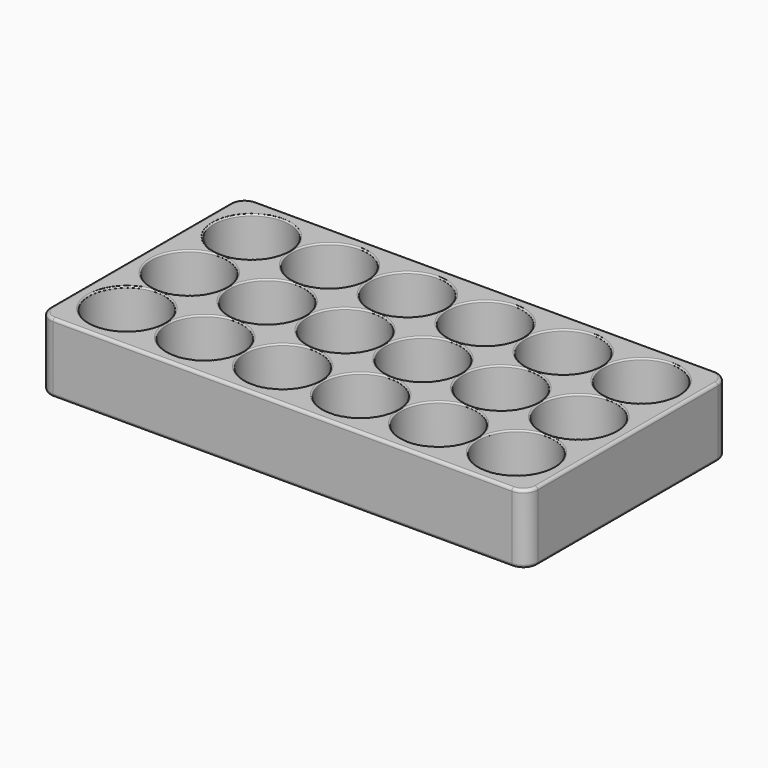
from build123d import *

# Parameters (mm, degrees)
F0_W         = 169
F0_H         = 88
F0_R         = 13.1
F1_DEPTH     = 22
F2_W         = 169
F2_H         = 88
F3_DEPTH     = 2
F4_R         = 1
F6_T1_DEPTH  = 24
F6_T4_ANGLE  = 90
F6_T6_ANGLE  = 90
F6_T8_ANGLE  = 90
F6_T10_ANGLE = 90
F6_T12_ANGLE = 90
F6_T14_ANGLE = 90
F6_T16_ANGLE = 90
F6_T18_ANGLE = 90


# Not quite as in the source:
# - a fillet or chamfer that OpenCascade refuses, or shapes differently, is made with other operations: its cross-section is extruded or revolved along the edge and cut away or added


with BuildPart() as f1:
    # F0 (on Top) → F1 (new body)
    with BuildSketch(Plane.XY):
        with Locations((67.5, 27)):
            Rectangle(F0_W, F0_H)
        Circle(F0_R, mode=Mode.SUBTRACT)
        with Locations((27, 0)):
            Circle(F0_R, mode=Mode.SUBTRACT)
        with Locations((54, 0)):
            Circle(F0_R, mode=Mode.SUBTRACT)
        with Locations((81, 0)):
            Circle(F0_R, mode=Mode.SUBTRACT)
        with Locations((108, 0)):
            Circle(F0_R, mode=Mode.SUBTRACT)
        with Locations((135, 0)):
            Circle(F0_R, mode=Mode.SUBTRACT)
        with Locations((0, 27)):
            Circle(F0_R, mode=Mode.SUBTRACT)
        with Locations((27, 27)):
            Circle(F0_R, mode=Mode.SUBTRACT)
        with Locations((54, 27)):
            Circle(F0_R, mode=Mode.SUBTRACT)
        with Locations((0, 54)):
            Circle(F0_R, mode=Mode.SUBTRACT)
        with Locations((27, 54)):
            Circle(F0_R, mode=Mode.SUBTRACT)
        with Locations((54, 54)):
            Circle(F0_R, mode=Mode.SUBTRACT)
        with Locations((81, 27)):
            Circle(F0_R, mode=Mode.SUBTRACT)
        with Locations((108, 27)):
            Circle(F0_R, mode=Mode.SUBTRACT)
        with Locations((135, 27)):
            Circle(F0_R, mode=Mode.SUBTRACT)
        with Locations((81, 54)):
            Circle(F0_R, mode=Mode.SUBTRACT)
        with Locations((108, 54)):
            Circle(F0_R, mode=Mode.SUBTRACT)
        with Locations((135, 54)):
            Circle(F0_R, mode=Mode.SUBTRACT)
    extrude(amount=-F1_DEPTH)

    # F2 (on face) → F3 (join)
    with BuildSketch(Plane(origin=(0, 0, -22), x_dir=(1, 0, 0), z_dir=(0, 0, -1))):
        with Locations((67.5, -27)):
            Rectangle(F2_W, F2_H)
    extrude(amount=F3_DEPTH)

    # F4
    f4_edges = [f1.edges().sort_by_distance(p)[0] for p in [
        (-17, 27, 0),
        (67.5, 71, 0),
        (152, 27, 0),
        (67.5, -17, 0),
        (67.5, 71, -24),
        (152, 27, -24),
        (67.5, -17, -24),
        (-17, 27, -24),
    ]]
    fillet(f4_edges, radius=F4_R)

    # F5: fillet of radius 0.5 on 22 edges, made by hand

    # F5_s1 → F5_t2 (revolve, cut)
    with BuildSketch(Plane.XZ):
        with BuildLine():
            ThreePointArc((148.6, 0), (148.2464466094, -0.1464466094), (148.1, -0.5))
            Line((148.1, -0.5), (148.1, 0))
            Line((148.1, 0), (148.6, 0))
        make_face()
    revolve(axis=Axis((135, 0, 0), (0, 0, 1)), mode=Mode.SUBTRACT)

    # F5_s3 → F5_t4 (revolve, cut)
    with BuildSketch(Plane.XZ):
        with BuildLine():
            ThreePointArc((13.6, 0), (13.2464466094, -0.1464466094), (13.1, -0.5))
            Line((13.1, -0.5), (13.1, 0))
            Line((13.1, 0), (13.6, 0))
        make_face()
    revolve(axis=Axis((0, 0, 0), (0, 0, 1)), mode=Mode.SUBTRACT)

    # F5_s5 → F5_t6 (revolve, cut)
    with BuildSketch(Plane.XZ):
        with BuildLine():
            ThreePointArc((40.6, 0), (40.2464466094, -0.1464466094), (40.1, -0.5))
            Line((40.1, -0.5), (40.1, 0))
            Line((40.1, 0), (40.6, 0))
        make_face()
    revolve(axis=Axis((27, 0, 0), (0, 0, 1)), mode=Mode.SUBTRACT)

    # F5_s7 → F5_t8 (revolve, cut)
    with BuildSketch(Plane.XZ):
        with BuildLine():
            ThreePointArc((67.6, 0), (67.2464466094, -0.1464466094), (67.1, -0.5))
            Line((67.1, -0.5), (67.1, 0))
            Line((67.1, 0), (67.6, 0))
        make_face()
    revolve(axis=Axis((54, 0, 0), (0, 0, 1)), mode=Mode.SUBTRACT)

    # F5_s9 → F5_t10 (revolve, cut)
    with BuildSketch(Plane.XZ):
        with BuildLine():
            ThreePointArc((94.6, 0), (94.2464466094, -0.1464466094), (94.1, -0.5))
            Line((94.1, -0.5), (94.1, 0))
            Line((94.1, 0), (94.6, 0))
        make_face()
    revolve(axis=Axis((81, 0, 0), (0, 0, 1)), mode=Mode.SUBTRACT)

    # F5_s11 → F5_t12 (revolve, cut)
    with BuildSketch(Plane.XZ):
        with BuildLine():
            ThreePointArc((121.6, 0), (121.2464466094, -0.1464466094), (121.1, -0.5))
            Line((121.1, -0.5), (121.1, 0))
            Line((121.1, 0), (121.6, 0))
        make_face()
    revolve(axis=Axis((108, 0, 0), (0, 0, 1)), mode=Mode.SUBTRACT)

    # F5_s13 → F5_t14 (revolve, cut)
    with BuildSketch(Plane.XZ.offset(-27)):
        with BuildLine():
            ThreePointArc((13.6, 0), (13.2464466094, -0.1464466094), (13.1, -0.5))
            Line((13.1, -0.5), (13.1, 0))
            Line((13.1, 0), (13.6, 0))
        make_face()
    revolve(axis=Axis((0, 27, 0), (0, 0, 1)), mode=Mode.SUBTRACT)

    # F5_s15 → F5_t16 (revolve, cut)
    with BuildSketch(Plane.XZ.offset(-27)):
        with BuildLine():
            ThreePointArc((40.6, 0), (40.2464466094, -0.1464466094), (40.1, -0.5))
            Line((40.1, -0.5), (40.1, 0))
            Line((40.1, 0), (40.6, 0))
        make_face()
    revolve(axis=Axis((27, 27, 0), (0, 0, 1)), mode=Mode.SUBTRACT)

    # F5_s17 → F5_t18 (revolve, cut)
    with BuildSketch(Plane.XZ.offset(-27)):
        with BuildLine():
            ThreePointArc((67.6, 0), (67.2464466094, -0.1464466094), (67.1, -0.5))
            Line((67.1, -0.5), (67.1, 0))
            Line((67.1, 0), (67.6, 0))
        make_face()
    revolve(axis=Axis((54, 27, 0), (0, 0, 1)), mode=Mode.SUBTRACT)

    # F5_s19 → F5_t20 (revolve, cut)
    with BuildSketch(Plane.XZ.offset(-54)):
        with BuildLine():
            ThreePointArc((13.6, 0), (13.2464466094, -0.1464466094), (13.1, -0.5))
            Line((13.1, -0.5), (13.1, 0))
            Line((13.1, 0), (13.6, 0))
        make_face()
    revolve(axis=Axis((0, 54, 0), (0, 0, 1)), mode=Mode.SUBTRACT)

    # F5_s21 → F5_t22 (revolve, cut)
    with BuildSketch(Plane.XZ.offset(-54)):
        with BuildLine():
            ThreePointArc((40.6, 0), (40.2464466094, -0.1464466094), (40.1, -0.5))
            Line((40.1, -0.5), (40.1, 0))
            Line((40.1, 0), (40.6, 0))
        make_face()
    revolve(axis=Axis((27, 54, 0), (0, 0, 1)), mode=Mode.SUBTRACT)

    # F5_s23 → F5_t24 (revolve, cut)
    with BuildSketch(Plane.XZ.offset(-54)):
        with BuildLine():
            ThreePointArc((67.6, 0), (67.2464466094, -0.1464466094), (67.1, -0.5))
            Line((67.1, -0.5), (67.1, 0))
            Line((67.1, 0), (67.6, 0))
        make_face()
    revolve(axis=Axis((54, 54, 0), (0, 0, 1)), mode=Mode.SUBTRACT)

    # F5_s25 → F5_t26 (revolve, cut)
    with BuildSketch(Plane.XZ.offset(-27)):
        with BuildLine():
            ThreePointArc((94.6, 0), (94.2464466094, -0.1464466094), (94.1, -0.5))
            Line((94.1, -0.5), (94.1, 0))
            Line((94.1, 0), (94.6, 0))
        make_face()
    revolve(axis=Axis((81, 27, 0), (0, 0, 1)), mode=Mode.SUBTRACT)

    # F5_s27 → F5_t28 (revolve, cut)
    with BuildSketch(Plane.XZ.offset(-27)):
        with BuildLine():
            ThreePointArc((121.6, 0), (121.2464466094, -0.1464466094), (121.1, -0.5))
            Line((121.1, -0.5), (121.1, 0))
            Line((121.1, 0), (121.6, 0))
        make_face()
    revolve(axis=Axis((108, 27, 0), (0, 0, 1)), mode=Mode.SUBTRACT)

    # F5_s29 → F5_t30 (revolve, cut)
    with BuildSketch(Plane.XZ.offset(-27)):
        with BuildLine():
            ThreePointArc((148.6, 0), (148.2464466094, -0.1464466094), (148.1, -0.5))
            Line((148.1, -0.5), (148.1, 0))
            Line((148.1, 0), (148.6, 0))
        make_face()
    revolve(axis=Axis((135, 27, 0), (0, 0, 1)), mode=Mode.SUBTRACT)

    # F5_s31 → F5_t32 (revolve, cut)
    with BuildSketch(Plane.XZ.offset(-54)):
        with BuildLine():
            ThreePointArc((94.6, 0), (94.2464466094, -0.1464466094), (94.1, -0.5))
            Line((94.1, -0.5), (94.1, 0))
            Line((94.1, 0), (94.6, 0))
        make_face()
    revolve(axis=Axis((81, 54, 0), (0, 0, 1)), mode=Mode.SUBTRACT)

    # F5_s33 → F5_t34 (revolve, cut)
    with BuildSketch(Plane.XZ.offset(-54)):
        with BuildLine():
            ThreePointArc((121.6, 0), (121.2464466094, -0.1464466094), (121.1, -0.5))
            Line((121.1, -0.5), (121.1, 0))
            Line((121.1, 0), (121.6, 0))
        make_face()
    revolve(axis=Axis((108, 54, 0), (0, 0, 1)), mode=Mode.SUBTRACT)

    # F5_s35 → F5_t36 (revolve, cut)
    with BuildSketch(Plane.XZ.offset(-54)):
        with BuildLine():
            ThreePointArc((148.6, 0), (148.2464466094, -0.1464466094), (148.1, -0.5))
            Line((148.1, -0.5), (148.1, 0))
            Line((148.1, 0), (148.6, 0))
        make_face()
    revolve(axis=Axis((135, 54, 0), (0, 0, 1)), mode=Mode.SUBTRACT)

    # F6: fillet of radius 5 on 4 edges, made by hand

    # F6_s2 → F6_t1 (cut)
    with BuildSketch(Plane.XY.offset(-24)):
        with BuildLine():
            ThreePointArc((-12, 71), (-15.5355339059, 69.5355339059), (-17, 66))
            Line((-17, 66), (-17, 71))
            Line((-17, 71), (-12, 71))
        make_face()
        with BuildLine():
            ThreePointArc((-17, -12), (-15.5355339059, -15.5355339059), (-12, -17))
            Line((-12, -17), (-17, -17))
            Line((-17, -17), (-17, -12))
        make_face()
        with BuildLine():
            ThreePointArc((147, 71), (150.5355339059, 69.5355339059), (152, 66))
            Line((152, 66), (152, 71))
            Line((152, 71), (147, 71))
        make_face()
        with BuildLine():
            ThreePointArc((152, -12), (150.5355339059, -15.5355339059), (147, -17))
            Line((147, -17), (152, -17))
            Line((152, -17), (152, -12))
        make_face()
    extrude(amount=F6_T1_DEPTH, mode=Mode.SUBTRACT)

    # F6_s3 → F6_t4 (revolve, cut)
    with BuildSketch(Plane.YZ.offset(147)):
        with BuildLine():
            ThreePointArc((-16, 0), (-16.7071067812, -0.2928932188), (-17, -1))
            Line((-17, -1), (-17, 0))
            Line((-17, 0), (-16, 0))
        make_face()
    revolve(axis=Axis((147, -12, 0), (0, 0, 1)), revolution_arc=F6_T4_ANGLE, mode=Mode.SUBTRACT)

    # F6_s5 → F6_t6 (revolve, cut)
    with BuildSketch(Plane.XZ.offset(12)):
        with BuildLine():
            ThreePointArc((151, -24), (151.7071067812, -23.7071067812), (152, -23))
            Line((152, -23), (152, -24))
            Line((152, -24), (151, -24))
        make_face()
    revolve(axis=Axis((147, -12, -24), (0, 0, -1)), revolution_arc=F6_T6_ANGLE, mode=Mode.SUBTRACT)

    # F6_s7 → F6_t8 (revolve, cut)
    with BuildSketch(Plane.XZ.offset(-66)):
        with BuildLine():
            ThreePointArc((151, 0), (151.7071067812, -0.2928932188), (152, -1))
            Line((152, -1), (152, 0))
            Line((152, 0), (151, 0))
        make_face()
    revolve(axis=Axis((147, 66, 0), (0, 0, 1)), revolution_arc=F6_T8_ANGLE, mode=Mode.SUBTRACT)

    # F6_s9 → F6_t10 (revolve, cut)
    with BuildSketch(Plane.YZ.offset(147)):
        with BuildLine():
            ThreePointArc((70, -24), (70.7071067812, -23.7071067812), (71, -23))
            Line((71, -23), (71, -24))
            Line((71, -24), (70, -24))
        make_face()
    revolve(axis=Axis((147, 66, -24), (0, 0, -1)), revolution_arc=F6_T10_ANGLE, mode=Mode.SUBTRACT)

    # F6_s11 → F6_t12 (revolve, cut)
    with BuildSketch(Plane.YZ.offset(-12)):
        with BuildLine():
            ThreePointArc((-16, -24), (-16.7071067812, -23.7071067812), (-17, -23))
            Line((-17, -23), (-17, -24))
            Line((-17, -24), (-16, -24))
        make_face()
    revolve(axis=Axis((-12, -12, -24), (0, 0, -1)), revolution_arc=F6_T12_ANGLE, mode=Mode.SUBTRACT)

    # F6_s13 → F6_t14 (revolve, cut)
    with BuildSketch(Plane.XZ.offset(12)):
        with BuildLine():
            ThreePointArc((-16, 0), (-16.7071067812, -0.2928932188), (-17, -1))
            Line((-17, -1), (-17, 0))
            Line((-17, 0), (-16, 0))
        make_face()
    revolve(axis=Axis((-12, -12, 0), (0, 0, 1)), revolution_arc=F6_T14_ANGLE, mode=Mode.SUBTRACT)

    # F6_s15 → F6_t16 (revolve, cut)
    with BuildSketch(Plane.XZ.offset(-66)):
        with BuildLine():
            ThreePointArc((-16, -24), (-16.7071067812, -23.7071067812), (-17, -23))
            Line((-17, -23), (-17, -24))
            Line((-17, -24), (-16, -24))
        make_face()
    revolve(axis=Axis((-12, 66, -24), (0, 0, -1)), revolution_arc=F6_T16_ANGLE, mode=Mode.SUBTRACT)

    # F6_s17 → F6_t18 (revolve, cut)
    with BuildSketch(Plane.YZ.offset(-12)):
        with BuildLine():
            ThreePointArc((70, 0), (70.7071067812, -0.2928932188), (71, -1))
            Line((71, -1), (71, 0))
            Line((71, 0), (70, 0))
        make_face()
    revolve(axis=Axis((-12, 66, 0), (0, 0, 1)), revolution_arc=F6_T18_ANGLE, mode=Mode.SUBTRACT)


solid = f1.part
